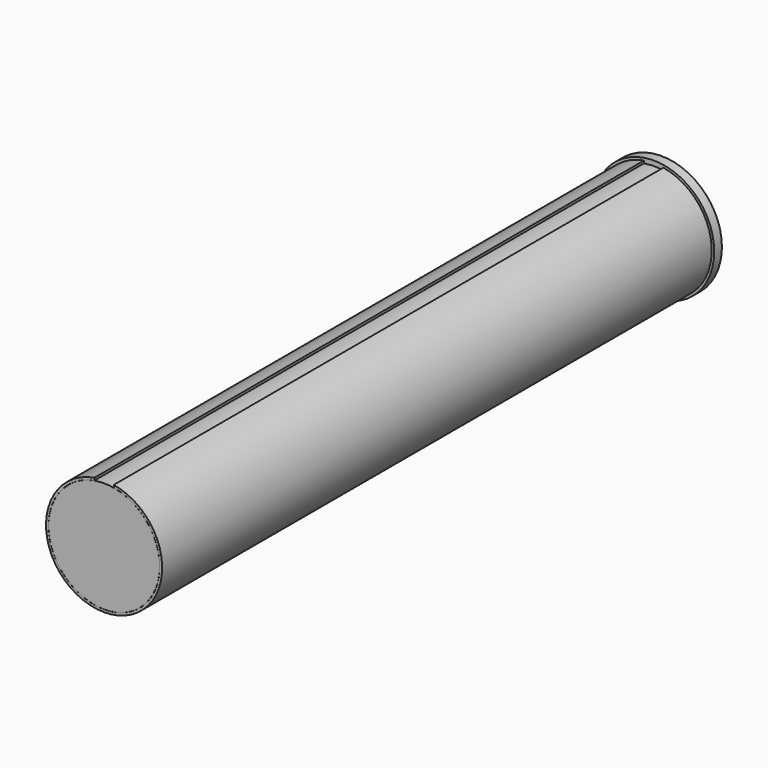
from build123d import *

# Parameters (mm, degrees)
F1_DEPTH      = 1828.8
F2_R          = 145.796
F3_DEPTH      = 1828.8
F4_R          = 18.7037822151
F5_DEPTH      = 152.401
F5_DEPTH_BACK = 150.2694264907
F6_R          = 158.75
F7_DEPTH      = 25.4
F8_R          = 21.9695909942
F9_DEPTH      = 254
F10_R         = 12.6554250347
F11_DEPTH     = 355.6


with BuildPart() as f1:
    # F0 (on Front) → F1 (new body)
    with BuildSketch(Plane.XZ):
        with BuildLine():
            Line((-25.4, 143.8243459919), (-25.4, 150.2684264907))
            ThreePointArc((-25.4, 150.2684264907), (0, -152.4), (25.4, 150.2684264907))
            Line((25.4, 150.2684264907), (25.4, 143.8243459919))
            ThreePointArc((25.4, 143.8243459919), (0, -146.05), (-25.4, 143.8243459919))
        make_face()
    extrude(amount=F1_DEPTH)


with BuildPart() as f3:
    # F2 (on Front) → F3 (new body)
    with BuildSketch(Plane.XZ):
        Circle(F2_R)
    extrude(amount=F3_DEPTH)

    # F4 (on Top) → F5 (cut, two sides)
    with BuildSketch(Plane.XY) as f5_sk:
        with Locations((63.4696483612, -76.1341750622)):
            Circle(F4_R)
    extrude(amount=-F5_DEPTH, mode=Mode.SUBTRACT)
    extrude(f5_sk.sketch, amount=F5_DEPTH_BACK, mode=Mode.SUBTRACT)

    # F8 (on Right) → F9 (cut)
    with BuildSketch(Plane.YZ):
        with Locations((-169.4504618645, 95.5888330936)):
            Circle(F8_R)
    extrude(amount=F9_DEPTH, mode=Mode.SUBTRACT)


with BuildPart() as f7:
    # F6 (on Front) → F7 (new body)
    with BuildSketch(Plane.XZ):
        Circle(F6_R)
    extrude(amount=F7_DEPTH)


with BuildPart() as f11_tool:
    # F10 (on Right) → F11 (new body)
    with BuildSketch(Plane.YZ):
        with Locations((-113.912537694, 0)):
            Circle(F10_R)
    extrude(amount=-F11_DEPTH)


with BuildPart() as f1_1:
    add(f1.part)

    # F11: cut by f11_tool
    add(f11_tool.part, mode=Mode.SUBTRACT)


with BuildPart() as f3_1:
    add(f3.part)

    # F11: cut by f11_tool
    add(f11_tool.part, mode=Mode.SUBTRACT)


solid = Compound([f7.part, f1_1.part, f3_1.part])
